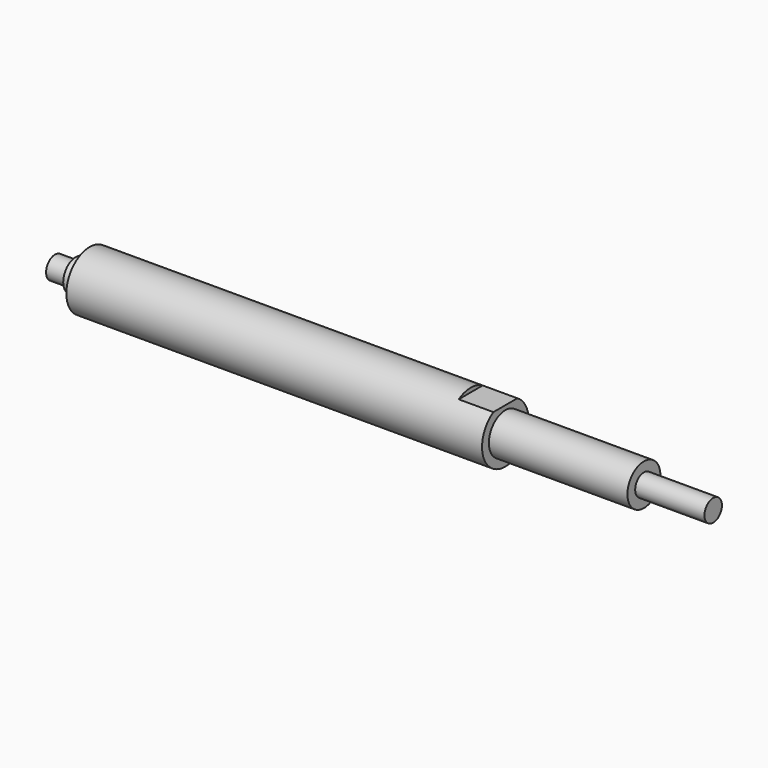
from build123d import *

# Parameters (mm, degrees)
F2_R     = 14.866691899
F3_DEPTH = 25


with BuildPart() as f1:
    # F0 (on Front) → F1 (revolve)
    with BuildSketch(Plane.XZ):
        Polygon((-116.810104717, 0), (358.189895283, 0), (358.189895283, 7.8803886721), (308.189895283, 7.8803886721), (308.189895283, 14.866691899), (208.189895283, 14.866691899), (208.189895283, 21.0310760423), (-91.810104717, 21.0310760423), (-91.810104717, 11.3735402855), (-101.810104717, 11.3735402855), (-101.810104717, 8.0858688513), (-116.810104717, 8.0858688513), align=None)
    revolve(axis=Axis((120.689895283, 0, 0), (1, 0, 0)))

    # F2 (on face) → F3 (cut)
    with BuildSketch(Plane.YZ.offset(208.189895283)):
        with BuildLine():
            Line((10.8252693386, 18.0310760423), (41.9066511095, 18.0310760423))
            Line((41.9066511095, 18.0310760423), (41.9066511095, 27.3393926871))
            Line((41.9066511095, 27.3393926871), (-41.9066511095, 27.3393926871))
            Line((-41.9066511095, 27.3393926871), (-41.9066511095, 18.0310760423))
            Line((-41.9066511095, 18.0310760423), (-10.8252693386, 18.0310760423))
            ThreePointArc((-10.8252693386, 18.0310760423), (0, 21.0310760423), (10.8252693386, 18.0310760423))
        make_face()
        with BuildLine():
            Line((-10.8252693386, 18.0310760423), (10.8252693386, 18.0310760423))
            ThreePointArc((10.8252693386, 18.0310760423), (0, 21.0310760423), (-10.8252693386, 18.0310760423))
        make_face()
        Circle(F2_R)
    extrude(amount=-F3_DEPTH, mode=Mode.SUBTRACT)


solid = f1.part
